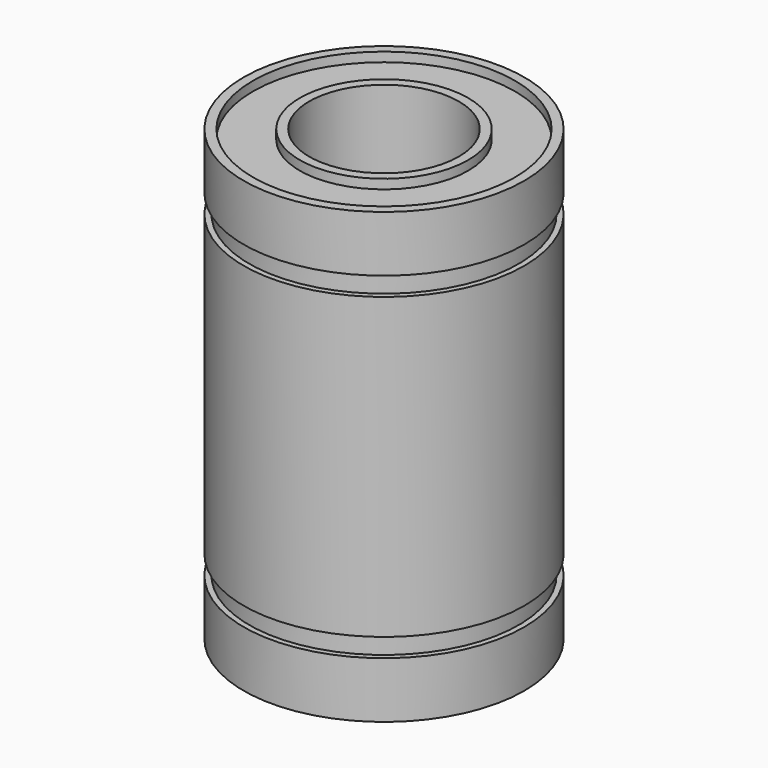
from build123d import *

# Parameters (mm, degrees)
F0_R     = 7.5
F0_R_2   = 4
F1_DEPTH = 24
F2_W     = 2.5912171826
F2_H     = 1
F4_R     = 7
F4_R_2   = 4.5
F5_DEPTH = 0.5


# Not quite as in the source:
# - a pattern or mirror of a feature is missing from the dataset's text; its kind, count and spacing are read off the source's solid


with BuildPart() as f1:
    # F0 (on Top) → F1 (new body)
    with BuildSketch(Plane.XY):
        Circle(F0_R)
        Circle(F0_R_2, mode=Mode.SUBTRACT)
    extrude(amount=F1_DEPTH)

    # F2 (on Right) → F3 (revolve, cut)
    with BuildSketch(Plane.YZ):
        with Locations((8.5017232858, 20.5)):
            Rectangle(F2_W, F2_H)
        with Locations((8.5017232858, 3.5)):
            Rectangle(F2_W, F2_H)
    revolve(axis=Axis((0, 0, 24), (0, 0, 1)), mode=Mode.SUBTRACT)

    # F4 (on face) → F5 (cut)
    with BuildSketch(Plane.XY.offset(24)):
        Circle(F4_R)
        Circle(F4_R_2, mode=Mode.SUBTRACT)
    f5 = extrude(amount=-F5_DEPTH, mode=Mode.SUBTRACT)

    # F5_copies: F5 across plane
    add(f5.mirror(Plane(origin=(0, 0, 12), x_dir=(-1, 0, 0), z_dir=(0, 0, -1))), mode=Mode.SUBTRACT)


solid = f1.part
